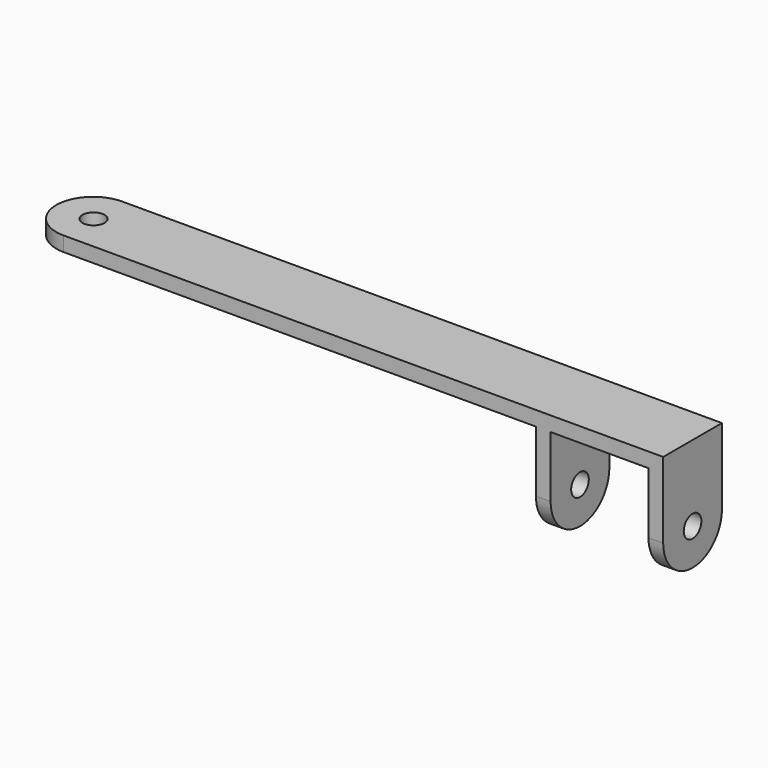
from build123d import *

# Parameters (mm, degrees)
F0_W     = 3
F0_H     = 20
F1_DEPTH = 15
F3_D     = 4.5
F3_DEPTH = 4
F3_TIP   = 1.3519363928
F5_D     = 4.5
F6_R     = 7.5
F7_R     = 7.49999


# Not quite as in the source:
# - a fillet or chamfer is up to 0.001 mm smaller than in the source, because OpenCascade refuses the exact size


with BuildPart() as f1:
    # F0 (on Front) → F1 (new body)
    with BuildSketch(Plane.XZ):
        with Locations((25.3187853247, -10)):
            Rectangle(F0_W, F0_H)
        with Locations((48.3187853247, -10)):
            Rectangle(F0_W, F0_H)
        Polygon((49.8187853247, 3), (-80.1812146753, 3), (-80.1812146753, 0), (23.8187853247, 0), (26.8187853247, 0), (46.8187853247, 0), (49.8187853247, 0), align=None)
    extrude(amount=F1_DEPTH)

    # F3
    with Locations(Plane(origin=(0, 0, 0), x_dir=(1, 0, 0), z_dir=(0, 0, -1))):
        with Locations((-72.5346971303, 7.5479238294)):
            Hole(F3_D / 2, depth=F3_DEPTH)
            with Locations((0, 0, -(F3_DEPTH + F3_TIP / 2))):  # 118° drill point
                Cone(0, F3_D / 2, F3_TIP, mode=Mode.SUBTRACT)

    # F5 (through all)
    with Locations(Plane.YZ.offset(49.8187853247)):
        with Locations((-7.5, -12.5)):
            Hole(F5_D / 2)

    # F6
    f6_edges = [f1.edges().sort_by_distance(p)[0] for p in [
        (48.318785, 0, -20),
    ]]
    fillet(f6_edges, radius=F6_R)

    # F7 (radius 7.5 in the source; OpenCascade refuses exactly that, so slightly less here)
    f7_edges = [f1.edges().sort_by_distance(p)[0] for p in [
        (25.318785, -15, -20),
        (48.318785, -15, -20),
        (25.318785, 0, -20),
        (-80.181215, 0, 1.5),
        (-80.181215, -15, 1.5),
    ]]
    fillet(f7_edges, radius=F7_R)


solid = f1.part
